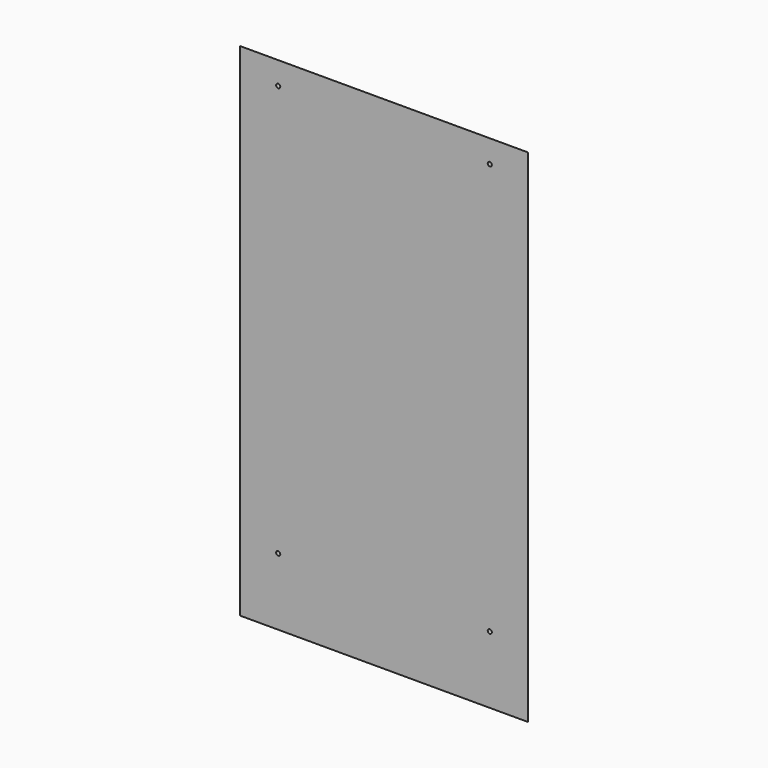
from build123d import *

# Parameters (mm, degrees)
F0_W     = 246
F0_H     = 429
F1_DEPTH = 12
F2_SIZE  = 11.99999
F4_D     = 3.5


# Not quite as in the source:
# - a fillet or chamfer is up to 0.001 mm smaller than in the source, because OpenCascade refuses the exact size
# - a feature names something its author has since deleted; it is built from what else it names


with BuildPart() as f1:
    # F0 (on Front) → F1 (new body)
    with BuildSketch(Plane.XZ):
        Rectangle(F0_W, F0_H)
    extrude(amount=F1_DEPTH)

    # F2 (size 12 in the source; OpenCascade refuses exactly that, so slightly less here)
    f2_edges = [f1.edges().sort_by_distance(p)[0] for p in [
        (123, 0, 0),
        (0, 0, 214.5),
        (-123, 0, 0),
    ]]
    chamfer(f2_edges, length=F2_SIZE)

    # F4 (through all)
    with Locations(Plane.XZ.offset(12)):
        with Locations((-90.5, 195), (90.5, 195), (-90.5, -157), (90.5, -157)):
            Hole(F4_D / 2)


solid = f1.part
